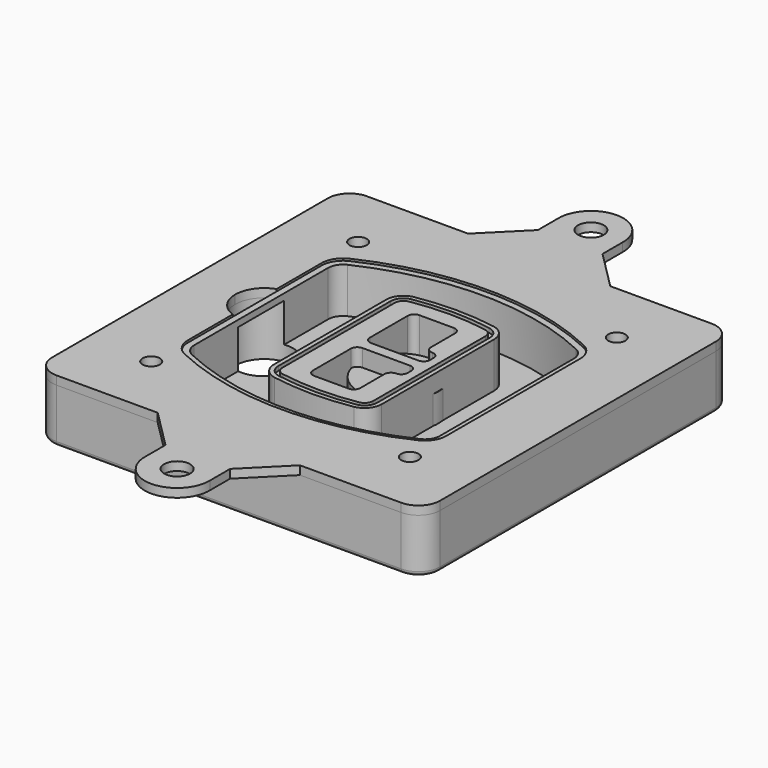
from build123d import *

# Parameters (mm, degrees)
F0_R      = 4
F1_DEPTH  = 25
F2_DEPTH  = 3
F3_DEPTH  = 18
F5_DEPTH  = 21
F6_DEPTH  = 2
F8_DEPTH  = 20
F9_DEPTH  = 16
F10_DEPTH = 25
F7_R      = 6
F7_R_2    = 4
F11_DEPTH = 6
F13_DEPTH = 9
F15_R     = 2
F16_R     = 6
F16_R_2   = 4
F17_DEPTH = 4


# Not quite as in the source:
# - a feature of the source that left no trace in its solid (it failed there, or was rolled back) is left out
# - a feature names something its author has since deleted; it is built from what else it names


with BuildPart() as f1:
    # F0 (on Top) → F1 (new body)
    with BuildSketch(Plane.XY):
        with BuildLine():
            ThreePointArc((-90, -80), (-87.0710678119, -87.0710678119), (-80, -90))
            Line((-80, -90), (80, -90))
            ThreePointArc((80, -90), (87.0710678119, -87.0710678119), (90, -80))
            Line((90, -80), (90, 80))
            ThreePointArc((90, 80), (87.0710678119, 87.0710678119), (80, 90))
            Line((80, 90), (-80, 90))
            ThreePointArc((-80, 90), (-87.0710678119, 87.0710678119), (-90, 80))
            Line((-90, 80), (-90, -80))
        make_face()
        with Locations((-60, -60)):
            Circle(F0_R, mode=Mode.SUBTRACT)
        with Locations((60, -60)):
            Circle(F0_R, mode=Mode.SUBTRACT)
        with BuildLine():
            ThreePointArc((-64, 38.8308515907), (-61.8195654598, 46.3340424013), (-55.9574468085, 51.5000594398))
            ThreePointArc((-55.9574468085, 51.5000594398), (0, 64), (55.9574468085, 51.5000594398))
            ThreePointArc((55.9574468085, 51.5000594398), (61.8195654598, 46.3340424013), (64, 38.8308515907))
            Line((64, 38.8308515907), (64, -38.8308515907))
            ThreePointArc((64, -38.8308515907), (61.8195654598, -46.3340424013), (55.9574468085, -51.5000594398))
            ThreePointArc((55.9574468085, -51.5000594398), (0, -64), (-55.9574468085, -51.5000594398))
            ThreePointArc((-55.9574468085, -51.5000594398), (-61.8195654598, -46.3340424013), (-64, -38.8308515907))
            Line((-64, -38.8308515907), (-64, 38.8308515907))
        make_face(mode=Mode.SUBTRACT)
        with Locations((-60, 60)):
            Circle(F0_R, mode=Mode.SUBTRACT)
        with Locations((60, 60)):
            Circle(F0_R, mode=Mode.SUBTRACT)
        with BuildLine():
            ThreePointArc((55.9574468085, 51.5000594398), (0, 64), (-55.9574468085, 51.5000594398))
            ThreePointArc((-55.9574468085, 51.5000594398), (-61.8195654598, 46.3340424013), (-64, 38.8308515907))
            Line((-64, 38.8308515907), (-64, -38.8308515907))
            ThreePointArc((-64, -38.8308515907), (-61.8195654598, -46.3340424013), (-55.9574468085, -51.5000594398))
            ThreePointArc((-55.9574468085, -51.5000594398), (0, -64), (55.9574468085, -51.5000594398))
            ThreePointArc((55.9574468085, -51.5000594398), (61.8195654598, -46.3340424013), (64, -38.8308515907))
            Line((64, -38.8308515907), (64, 38.8308515907))
            ThreePointArc((64, 38.8308515907), (61.8195654598, 46.3340424013), (55.9574468085, 51.5000594398))
        make_face()
        with BuildLine():
            Line((-60, -38.8308515907), (-60, 38.8308515907))
            ThreePointArc((-60, 38.8308515907), (-58.442546757, 44.1902735983), (-54.2553191489, 47.8802857686))
            ThreePointArc((-54.2553191489, 47.8802857686), (0, 60), (54.2553191489, 47.8802857686))
            ThreePointArc((54.2553191489, 47.8802857686), (58.442546757, 44.1902735983), (60, 38.8308515907))
            Line((60, 38.8308515907), (60, -38.8308515907))
            ThreePointArc((60, -38.8308515907), (58.442546757, -44.1902735983), (54.2553191489, -47.8802857686))
            ThreePointArc((54.2553191489, -47.8802857686), (0, -60), (-54.2553191489, -47.8802857686))
            ThreePointArc((-54.2553191489, -47.8802857686), (-58.442546757, -44.1902735983), (-60, -38.8308515907))
        make_face(mode=Mode.SUBTRACT)
        with BuildLine():
            ThreePointArc((-54.2553191489, 47.8802857686), (-58.442546757, 44.1902735983), (-60, 38.8308515907))
            Line((-60, 38.8308515907), (-60, -38.8308515907))
            ThreePointArc((-60, -38.8308515907), (-58.442546757, -44.1902735983), (-54.2553191489, -47.8802857686))
            ThreePointArc((-54.2553191489, -47.8802857686), (0, -60), (54.2553191489, -47.8802857686))
            ThreePointArc((54.2553191489, -47.8802857686), (58.442546757, -44.1902735983), (60, -38.8308515907))
            Line((60, -38.8308515907), (60, 38.8308515907))
            ThreePointArc((60, 38.8308515907), (58.442546757, 44.1902735983), (54.2553191489, 47.8802857686))
            ThreePointArc((54.2553191489, 47.8802857686), (0, 60), (-54.2553191489, 47.8802857686))
        make_face()
        with BuildLine():
            ThreePointArc((52.9787234043, 45.1654555152), (55.9097827299, 42.582446996), (57, 38.8308515907))
            Line((57, 38.8308515907), (57, -38.8308515907))
            ThreePointArc((57, -38.8308515907), (55.9097827299, -42.582446996), (52.9787234043, -45.1654555152))
            ThreePointArc((52.9787234043, -45.1654555152), (0, -57), (-52.9787234043, -45.1654555152))
            ThreePointArc((-52.9787234043, -45.1654555152), (-55.9097827299, -42.582446996), (-57, -38.8308515907))
            Line((-57, -38.8308515907), (-57, 38.8308515907))
            ThreePointArc((-57, 38.8308515907), (-55.9097827299, 42.582446996), (-52.9787234043, 45.1654555152))
            ThreePointArc((-52.9787234043, 45.1654555152), (0, 57), (52.9787234043, 45.1654555152))
        make_face(mode=Mode.SUBTRACT)
        with BuildLine():
            Line((57, -38.8308515907), (57, 38.8308515907))
            ThreePointArc((57, 38.8308515907), (55.9097827299, 42.582446996), (52.9787234043, 45.1654555152))
            ThreePointArc((52.9787234043, 45.1654555152), (0, 57), (-52.9787234043, 45.1654555152))
            ThreePointArc((-52.9787234043, 45.1654555152), (-55.9097827299, 42.582446996), (-57, 38.8308515907))
            Line((-57, 38.8308515907), (-57, -38.8308515907))
            ThreePointArc((-57, -38.8308515907), (-55.9097827299, -42.582446996), (-52.9787234043, -45.1654555152))
            ThreePointArc((-52.9787234043, -45.1654555152), (0, -57), (52.9787234043, -45.1654555152))
            ThreePointArc((52.9787234043, -45.1654555152), (55.9097827299, -42.582446996), (57, -38.8308515907))
        make_face()
    extrude(amount=-F1_DEPTH)

    # F0 (on Top) → F2 (join)
    with BuildSketch(Plane.XY):
        with BuildLine():
            ThreePointArc((-54.2553191489, 47.8802857686), (-58.442546757, 44.1902735983), (-60, 38.8308515907))
            Line((-60, 38.8308515907), (-60, -38.8308515907))
            ThreePointArc((-60, -38.8308515907), (-58.442546757, -44.1902735983), (-54.2553191489, -47.8802857686))
            ThreePointArc((-54.2553191489, -47.8802857686), (0, -60), (54.2553191489, -47.8802857686))
            ThreePointArc((54.2553191489, -47.8802857686), (58.442546757, -44.1902735983), (60, -38.8308515907))
            Line((60, -38.8308515907), (60, 38.8308515907))
            ThreePointArc((60, 38.8308515907), (58.442546757, 44.1902735983), (54.2553191489, 47.8802857686))
            ThreePointArc((54.2553191489, 47.8802857686), (0, 60), (-54.2553191489, 47.8802857686))
        make_face()
        with BuildLine():
            ThreePointArc((52.9787234043, 45.1654555152), (55.9097827299, 42.582446996), (57, 38.8308515907))
            Line((57, 38.8308515907), (57, -38.8308515907))
            ThreePointArc((57, -38.8308515907), (55.9097827299, -42.582446996), (52.9787234043, -45.1654555152))
            ThreePointArc((52.9787234043, -45.1654555152), (0, -57), (-52.9787234043, -45.1654555152))
            ThreePointArc((-52.9787234043, -45.1654555152), (-55.9097827299, -42.582446996), (-57, -38.8308515907))
            Line((-57, -38.8308515907), (-57, 38.8308515907))
            ThreePointArc((-57, 38.8308515907), (-55.9097827299, 42.582446996), (-52.9787234043, 45.1654555152))
            ThreePointArc((-52.9787234043, 45.1654555152), (0, 57), (52.9787234043, 45.1654555152))
        make_face(mode=Mode.SUBTRACT)
    extrude(amount=F2_DEPTH)

    # F0 (on Top) → F3 (cut)
    with BuildSketch(Plane.XY):
        with BuildLine():
            Line((57, -38.8308515907), (57, 38.8308515907))
            ThreePointArc((57, 38.8308515907), (55.9097827299, 42.582446996), (52.9787234043, 45.1654555152))
            ThreePointArc((52.9787234043, 45.1654555152), (0, 57), (-52.9787234043, 45.1654555152))
            ThreePointArc((-52.9787234043, 45.1654555152), (-55.9097827299, 42.582446996), (-57, 38.8308515907))
            Line((-57, 38.8308515907), (-57, -38.8308515907))
            ThreePointArc((-57, -38.8308515907), (-55.9097827299, -42.582446996), (-52.9787234043, -45.1654555152))
            ThreePointArc((-52.9787234043, -45.1654555152), (0, -57), (52.9787234043, -45.1654555152))
            ThreePointArc((52.9787234043, -45.1654555152), (55.9097827299, -42.582446996), (57, -38.8308515907))
        make_face()
    extrude(amount=-F3_DEPTH, mode=Mode.SUBTRACT)

    # F4 (on face) → F5 (join, through all)
    with BuildSketch(Plane.XY.offset(3)):
        with BuildLine():
            ThreePointArc((-25, -32.5662280692), (-23.1122504785, -37.7276614059), (-18.3399014778, -40.4532214146))
            ThreePointArc((-18.3399014778, -40.4532214146), (0, -42), (18.3399014778, -40.4532214146))
            ThreePointArc((18.3399014778, -40.4532214146), (23.1122504785, -37.7276614059), (25, -32.5662280692))
            Line((25, -32.5662280692), (25, 32.5662280692))
            ThreePointArc((25, 32.5662280692), (23.1122504785, 37.7276614059), (18.3399014778, 40.4532214146))
            ThreePointArc((18.3399014778, 40.4532214146), (0, 42), (-18.3399014778, 40.4532214146))
            ThreePointArc((-18.3399014778, 40.4532214146), (-23.1122504785, 37.7276614059), (-25, 32.5662280692))
            Line((-25, 32.5662280692), (-25, -32.5662280692))
        make_face()
        with BuildLine():
            ThreePointArc((18.0049261084, 38.4814730782), (21.5841878588, 36.4373030717), (23, 32.5662280692))
            Line((23, 32.5662280692), (23, -32.5662280692))
            ThreePointArc((23, -32.5662280692), (21.5841878588, -36.4373030717), (18.0049261084, -38.4814730782))
            ThreePointArc((18.0049261084, -38.4814730782), (0, -40), (-18.0049261084, -38.4814730782))
            ThreePointArc((-18.0049261084, -38.4814730782), (-21.5841878588, -36.4373030717), (-23, -32.5662280692))
            Line((-23, -32.5662280692), (-23, 32.5662280692))
            ThreePointArc((-23, 32.5662280692), (-21.5841878588, 36.4373030717), (-18.0049261084, 38.4814730782))
            ThreePointArc((-18.0049261084, 38.4814730782), (0, 40), (18.0049261084, 38.4814730782))
        make_face(mode=Mode.SUBTRACT)
        with BuildLine():
            Line((23, -32.5662280692), (23, 32.5662280692))
            ThreePointArc((23, 32.5662280692), (21.5841878588, 36.4373030717), (18.0049261084, 38.4814730782))
            ThreePointArc((18.0049261084, 38.4814730782), (0, 40), (-18.0049261084, 38.4814730782))
            ThreePointArc((-18.0049261084, 38.4814730782), (-21.5841878588, 36.4373030717), (-23, 32.5662280692))
            Line((-23, 32.5662280692), (-23, -32.5662280692))
            ThreePointArc((-23, -32.5662280692), (-21.5841878588, -36.4373030717), (-18.0049261084, -38.4814730782))
            ThreePointArc((-18.0049261084, -38.4814730782), (0, -40), (18.0049261084, -38.4814730782))
            ThreePointArc((18.0049261084, -38.4814730782), (21.5841878588, -36.4373030717), (23, -32.5662280692))
        make_face()
        with BuildLine():
            ThreePointArc((17.6699507389, 36.5097247419), (20.0561252392, 35.1469447375), (21, 32.5662280692))
            Line((21, 32.5662280692), (21, -32.5662280692))
            ThreePointArc((21, -32.5662280692), (20.0561252392, -35.1469447375), (17.6699507389, -36.5097247419))
            ThreePointArc((17.6699507389, -36.5097247419), (0, -38), (-17.6699507389, -36.5097247419))
            ThreePointArc((-17.6699507389, -36.5097247419), (-20.0561252392, -35.1469447375), (-21, -32.5662280692))
            Line((-21, -32.5662280692), (-21, 32.5662280692))
            ThreePointArc((-21, 32.5662280692), (-20.0561252392, 35.1469447375), (-17.6699507389, 36.5097247419))
            ThreePointArc((-17.6699507389, 36.5097247419), (0, 38), (17.6699507389, 36.5097247419))
        make_face(mode=Mode.SUBTRACT)
        with BuildLine():
            Line((21, -32.5662280692), (21, 32.5662280692))
            ThreePointArc((21, 32.5662280692), (20.0561252392, 35.1469447375), (17.6699507389, 36.5097247419))
            ThreePointArc((17.6699507389, 36.5097247419), (0, 38), (-17.6699507389, 36.5097247419))
            ThreePointArc((-17.6699507389, 36.5097247419), (-20.0561252392, 35.1469447375), (-21, 32.5662280692))
            Line((-21, 32.5662280692), (-21, -32.5662280692))
            ThreePointArc((-21, -32.5662280692), (-20.0561252392, -35.1469447375), (-17.6699507389, -36.5097247419))
            ThreePointArc((-17.6699507389, -36.5097247419), (0, -38), (17.6699507389, -36.5097247419))
            ThreePointArc((17.6699507389, -36.5097247419), (20.0561252392, -35.1469447375), (21, -32.5662280692))
        make_face()
        with BuildLine():
            Line((-8, -2.5), (14, -2.5))
            ThreePointArc((14, -2.5), (16.1213203436, -3.3786796564), (17, -5.5))
            Line((17, -5.5), (17, -7.5))
            ThreePointArc((17, -7.5), (16.1213203436, -9.6213203436), (14, -10.5))
            ThreePointArc((14, -10.5), (11.8786796564, -11.3786796564), (11, -13.5))
            Line((11, -13.5), (11, -27.5))
            ThreePointArc((11, -27.5), (10.1213203436, -29.6213203436), (8, -30.5))
            Line((8, -30.5), (-8, -30.5))
            ThreePointArc((-8, -30.5), (-10.1213203436, -29.6213203436), (-11, -27.5))
            Line((-11, -27.5), (-11, -5.5))
            ThreePointArc((-11, -5.5), (-10.1213203436, -3.3786796564), (-8, -2.5))
        make_face(mode=Mode.SUBTRACT)
        with BuildLine():
            ThreePointArc((-8, 2.5), (-10.1213203436, 3.3786796564), (-11, 5.5))
            Line((-11, 5.5), (-11, 27.5))
            ThreePointArc((-11, 27.5), (-10.1213203436, 29.6213203436), (-8, 30.5))
            Line((-8, 30.5), (8, 30.5))
            ThreePointArc((8, 30.5), (10.1213203436, 29.6213203436), (11, 27.5))
            Line((11, 27.5), (11, 13.5))
            ThreePointArc((11, 13.5), (11.8786796564, 11.3786796564), (14, 10.5))
            ThreePointArc((14, 10.5), (16.1213203436, 9.6213203436), (17, 7.5))
            Line((17, 7.5), (17, 5.5))
            ThreePointArc((17, 5.5), (16.1213203436, 3.3786796564), (14, 2.5))
            Line((14, 2.5), (-8, 2.5))
        make_face(mode=Mode.SUBTRACT)
    extrude(amount=-F5_DEPTH)

    # F4 (on face) → F6 (cut)
    with BuildSketch(Plane.XY.offset(3)):
        with BuildLine():
            Line((23, -32.5662280692), (23, 32.5662280692))
            ThreePointArc((23, 32.5662280692), (21.5841878588, 36.4373030717), (18.0049261084, 38.4814730782))
            ThreePointArc((18.0049261084, 38.4814730782), (0, 40), (-18.0049261084, 38.4814730782))
            ThreePointArc((-18.0049261084, 38.4814730782), (-21.5841878588, 36.4373030717), (-23, 32.5662280692))
            Line((-23, 32.5662280692), (-23, -32.5662280692))
            ThreePointArc((-23, -32.5662280692), (-21.5841878588, -36.4373030717), (-18.0049261084, -38.4814730782))
            ThreePointArc((-18.0049261084, -38.4814730782), (0, -40), (18.0049261084, -38.4814730782))
            ThreePointArc((18.0049261084, -38.4814730782), (21.5841878588, -36.4373030717), (23, -32.5662280692))
        make_face()
        with BuildLine():
            ThreePointArc((17.6699507389, 36.5097247419), (20.0561252392, 35.1469447375), (21, 32.5662280692))
            Line((21, 32.5662280692), (21, -32.5662280692))
            ThreePointArc((21, -32.5662280692), (20.0561252392, -35.1469447375), (17.6699507389, -36.5097247419))
            ThreePointArc((17.6699507389, -36.5097247419), (0, -38), (-17.6699507389, -36.5097247419))
            ThreePointArc((-17.6699507389, -36.5097247419), (-20.0561252392, -35.1469447375), (-21, -32.5662280692))
            Line((-21, -32.5662280692), (-21, 32.5662280692))
            ThreePointArc((-21, 32.5662280692), (-20.0561252392, 35.1469447375), (-17.6699507389, 36.5097247419))
            ThreePointArc((-17.6699507389, 36.5097247419), (0, 38), (17.6699507389, 36.5097247419))
        make_face(mode=Mode.SUBTRACT)
    extrude(amount=-F6_DEPTH, mode=Mode.SUBTRACT)

    # F7 (on face) → F8 (join)
    with BuildSketch(Plane(origin=(0, 0, -25), x_dir=(1, 0, 0), z_dir=(0, 0, -1))):
        with BuildLine():
            ThreePointArc((-6.71157564, 0), (6.7567035675, 13.4682792075), (20.224982775, 0))
            Line((20.224982775, 0), (25.224982775, 0))
            ThreePointArc((25.224982775, 0), (6.7567035675, 18.4682792075), (-11.71157564, 0))
            Line((-11.71157564, 0), (-6.71157564, 0))
        make_face()
        with BuildLine():
            Line((-6.71157564, 0), (20.224982775, 0))
            ThreePointArc((20.224982775, 0), (6.7567035675, 13.4682792075), (-6.71157564, 0))
        make_face()
        with BuildLine():
            ThreePointArc((-6.71157564, 0), (6.7567035675, -13.4682792075), (20.224982775, 0))
            Line((20.224982775, 0), (-6.71157564, 0))
        make_face()
        with BuildLine():
            Line((25.224982775, 0), (20.224982775, 0))
            ThreePointArc((20.224982775, 0), (6.7567035675, -13.4682792075), (-6.71157564, 0))
            Line((-6.71157564, 0), (-11.71157564, 0))
            ThreePointArc((-11.71157564, 0), (6.7567035675, -18.4682792075), (25.224982775, 0))
        make_face()
    extrude(amount=-F8_DEPTH)

    # F7 (on face) → F9 (cut)
    with BuildSketch(Plane(origin=(0, 0, -25), x_dir=(1, 0, 0), z_dir=(0, 0, -1))):
        with BuildLine():
            Line((-6.71157564, 0), (20.224982775, 0))
            ThreePointArc((20.224982775, 0), (6.7567035675, 13.4682792075), (-6.71157564, 0))
        make_face()
        with BuildLine():
            ThreePointArc((-6.71157564, 0), (6.7567035675, -13.4682792075), (20.224982775, 0))
            Line((20.224982775, 0), (-6.71157564, 0))
        make_face()
    extrude(amount=-F9_DEPTH, mode=Mode.SUBTRACT)

    # F7 (on face) → F10 (cut)
    with BuildSketch(Plane(origin=(0, 0, -25), x_dir=(1, 0, 0), z_dir=(0, 0, -1))):
        with BuildLine():
            Line((-69.0318229325, 0), (-42.0952645175, 0))
            ThreePointArc((-42.0952645175, 0), (-55.563543725, 13.4682792075), (-69.0318229325, 0))
        make_face()
        with BuildLine():
            ThreePointArc((-69.0318229325, 0), (-55.563543725, -13.4682792075), (-42.0952645175, 0))
            Line((-42.0952645175, 0), (-69.0318229325, 0))
        make_face()
    extrude(amount=-F10_DEPTH, mode=Mode.SUBTRACT)

    # F7 (on face) → F11 (cut)
    with BuildSketch(Plane(origin=(0, 0, -25), x_dir=(1, 0, 0), z_dir=(0, 0, -1))):
        with Locations((60, -60)):
            Circle(F7_R)
        with Locations((60, -60)):
            Circle(F7_R_2, mode=Mode.SUBTRACT)
        with Locations((-60, -60)):
            Circle(F7_R)
        with Locations((-60, -60)):
            Circle(F7_R_2, mode=Mode.SUBTRACT)
        with Locations((-60, 60)):
            Circle(F7_R)
        with Locations((-60, 60)):
            Circle(F7_R_2, mode=Mode.SUBTRACT)
        with Locations((60, 60)):
            Circle(F7_R)
        with Locations((60, 60)):
            Circle(F7_R_2, mode=Mode.SUBTRACT)
    extrude(amount=-F11_DEPTH, mode=Mode.SUBTRACT)

    # F12 (on face) → F13 (cut, through all)
    with BuildSketch(Plane(origin=(0, 0, -9), x_dir=(1, 0, 0), z_dir=(0, 0, -1))):
        with BuildLine():
            ThreePointArc((20.224982775, 0), (20.1663399806, 1.2554664788), (19.9909222755, 2.5))
            Line((19.9909222755, 2.5), (14, 2.5))
            ThreePointArc((14, 2.5), (16.1213203436, 3.3786796564), (17, 5.5))
            Line((17, 5.5), (17, 7.5))
            ThreePointArc((17, 7.5), (16.1213203436, 9.6213203436), (14, 10.5))
            ThreePointArc((14, 10.5), (12.1627255951, 11.1284134507), (11.0951631559, 12.750384826))
            ThreePointArc((11.0951631559, 12.750384826), (11.0476113807, 12.7664660322), (11, 12.7823698976))
            Line((11, 12.7823698976), (11, -12.7823698976))
            ThreePointArc((11, -12.7823698976), (11.0476113807, -12.7664660322), (11.0951631559, -12.750384826))
            ThreePointArc((11.0951631559, -12.750384826), (12.1627255951, -11.1284134507), (14, -10.5))
            ThreePointArc((14, -10.5), (16.1213203436, -9.6213203436), (17, -7.5))
            Line((17, -7.5), (17, -5.5))
            ThreePointArc((17, -5.5), (16.1213203436, -3.3786796564), (14, -2.5))
            Line((14, -2.5), (19.9909222755, -2.5))
            ThreePointArc((19.9909222755, -2.5), (20.1663399806, -1.2554664788), (20.224982775, 0))
        make_face()
    extrude(amount=F13_DEPTH, mode=Mode.SUBTRACT)

    # F15
    f15_edges = [f1.edges().sort_by_distance(p)[0] for p in [
        (0, -90, -25),
        (-87.071068, -87.071068, -25),
        (-90, 0, -25),
        (-87.071068, 87.071068, -25),
        (87.071068, -87.071068, -25),
        (0, 90, -25),
        (90, 0, -25),
        (87.071068, 87.071068, -25),
    ]]
    fillet(f15_edges, radius=F15_R)


with BuildPart() as f17:
    # F16 (on face) → F17 (new body)
    with BuildSketch(Plane.XY):
        with BuildLine():
            Line((-14.9930099735, 119.5421223602), (-14.9930099735, 108))
            Line((-14.9930099735, 108), (-32.9930099735, 90))
            Line((-32.9930099735, 90), (32.9930099735, 90))
            Line((32.9930099735, 90), (14.9930099735, 108))
            Line((14.9930099735, 108), (14.9930099735, 119.5421223602))
            ThreePointArc((14.9930099735, 119.5421223602), (0, 135), (-14.9930099735, 119.5421223602))
        make_face()
        with Locations((0, 120)):
            Circle(F16_R, mode=Mode.SUBTRACT)
        with BuildLine():
            Line((32.9930099735, 90), (-32.9930099735, 90))
            Line((-32.9930099735, 90), (-80, 90))
            ThreePointArc((-80, 90), (-87.0710678119, 87.0710678119), (-90, 80))
            Line((-90, 80), (-90, -80))
            ThreePointArc((-90, -80), (-87.0710678119, -87.0710678119), (-80, -90))
            Line((-80, -90), (-32.9930099735, -90))
            Line((-32.9930099735, -90), (32.9930099735, -90))
            Line((32.9930099735, -90), (80, -90))
            ThreePointArc((80, -90), (87.0710678119, -87.0710678119), (90, -80))
            Line((90, -80), (90, 80))
            ThreePointArc((90, 80), (87.0710678119, 87.0710678119), (80, 90))
            Line((80, 90), (32.9930099735, 90))
        make_face()
        with Locations((-60, -60)):
            Circle(F16_R_2, mode=Mode.SUBTRACT)
        with Locations((60, -60)):
            Circle(F16_R_2, mode=Mode.SUBTRACT)
        with Locations((-60, 60)):
            Circle(F16_R_2, mode=Mode.SUBTRACT)
        with BuildLine():
            ThreePointArc((-60, 38.8308515907), (-58.442546757, 44.1902735983), (-54.2553191489, 47.8802857686))
            ThreePointArc((-54.2553191489, 47.8802857686), (0, 60), (54.2553191489, 47.8802857686))
            ThreePointArc((54.2553191489, 47.8802857686), (58.442546757, 44.1902735983), (60, 38.8308515907))
            Line((60, 38.8308515907), (60, -38.8308515907))
            ThreePointArc((60, -38.8308515907), (58.442546757, -44.1902735983), (54.2553191489, -47.8802857686))
            ThreePointArc((54.2553191489, -47.8802857686), (0, -60), (-54.2553191489, -47.8802857686))
            ThreePointArc((-54.2553191489, -47.8802857686), (-58.442546757, -44.1902735983), (-60, -38.8308515907))
            Line((-60, -38.8308515907), (-60, -12.7166190685))
            ThreePointArc((-60, -12.7166190685), (-66.5441169481, -7.798817635), (-69.0318229325, 0))
            ThreePointArc((-69.0318229325, 0), (-66.5441169481, 7.798817635), (-60, 12.7166190685))
            Line((-60, 12.7166190685), (-60, 38.8308515907))
        make_face(mode=Mode.SUBTRACT)
        with Locations((60, 60)):
            Circle(F16_R_2, mode=Mode.SUBTRACT)
        with BuildLine():
            Line((32.9930099735, -90), (-32.9930099735, -90))
            Line((-32.9930099735, -90), (-14.9930099735, -108))
            Line((-14.9930099735, -108), (-14.9930099735, -119.5421223602))
            ThreePointArc((-14.9930099735, -119.5421223602), (0, -135), (14.9930099735, -119.5421223602))
            Line((14.9930099735, -119.5421223602), (14.9930099735, -108))
            Line((14.9930099735, -108), (32.9930099735, -90))
        make_face()
        with Locations((0, -120)):
            Circle(F16_R, mode=Mode.SUBTRACT)
    extrude(amount=F17_DEPTH)


solid = Compound([f1.part, f17.part])
